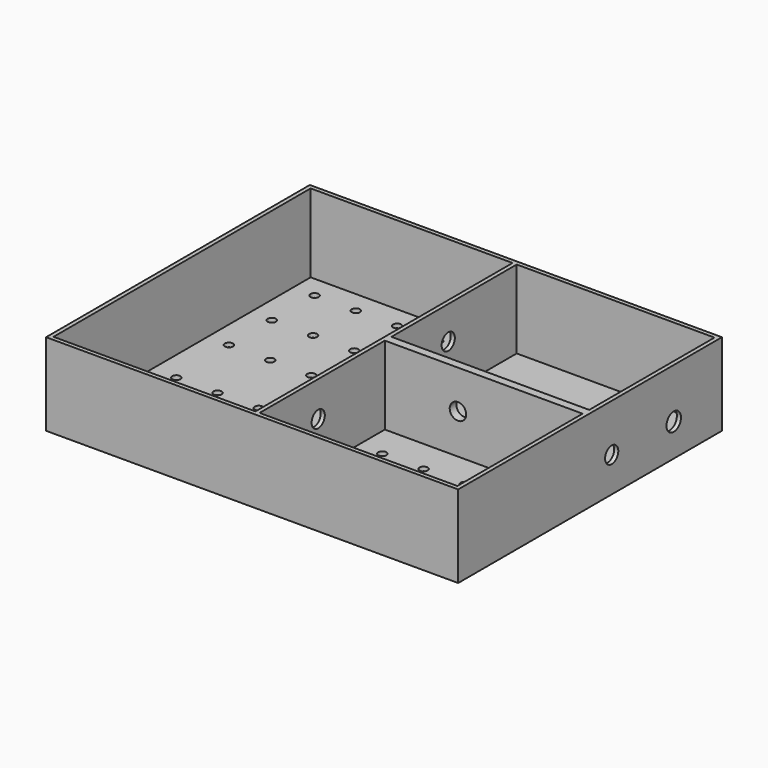
from build123d import *

# Parameters (mm, degrees)
F0_W      = 250
F0_H      = 200
F1_DEPTH  = 100
F2_T      = -5
F3_DEPTH  = 100
F4_T      = -5
F5_DEPTH  = 100
F6_T      = -5
F8_R      = 10
F9_DEPTH  = 25
F11_R     = 10
F12_DEPTH = 25
F14_R     = 5
F15_DEPTH = 25
F17_R     = 10
F18_DEPTH = 25
F19_R     = 11
F20_DEPTH = 25


# Not quite as in the source:
# - a shell that OpenCascade refuses in one call is made with other operations: the cavity is built on its own and cut out


with BuildPart() as f1:
    # F0 (on Top) → F1 (new body)
    with BuildSketch(Plane.XY):
        with Locations((375, -300)):
            Rectangle(F0_W, F0_H)
    extrude(amount=F1_DEPTH)

    # F2
    f2_openings = [f1.faces().sort_by_distance(p)[0] for p in [
        (375, -300, 100),
    ]]
    offset(amount=F2_T, openings=f2_openings)



with BuildPart() as f3:
    # F0 (on Top) → F3 (new body)
    with BuildSketch(Plane.XY):
        with Locations((375, -100)):
            Rectangle(F0_W, F0_H)
    extrude(amount=F3_DEPTH)

    # F4
    f4_openings = [f3.faces().sort_by_distance(p)[0] for p in [
        (375, -100, 100),
    ]]
    offset(amount=F4_T, openings=f4_openings)


with BuildPart() as f1_1:
    add(f1.part)

    add(f3.part)  # F5 merges F3
    # F0 (on Top) → F5 (join)
    with BuildSketch(Plane.XY):
        Polygon((250, 0), (0, 0), (0, -400), (250, -400), (250, -200), align=None)
    extrude(amount=F5_DEPTH)

    # F6: a shell. OpenCascade refuses it in one call, so the cavity is built on its own and cut out:
    # the body offset inwards by the wall thickness, plus a prism from it out through each open face.
    f6_core = offset(f1_1.part, amount=F6_T, kind=Kind.INTERSECTION, mode=Mode.PRIVATE)
    f6_exits = [f6_core.faces().sort_by_distance(p)[0] for p in [
        (127.5, -200, 95),
    ]]
    add(f6_core, mode=Mode.SUBTRACT)
    extrude(f6_exits, amount=-F6_T, mode=Mode.SUBTRACT)

    # F8 (on offset) → F9 (cut)
    with BuildSketch(Plane.YZ.offset(255)):
        with Locations((-108.8187620044, 59.8489716649)):
            Circle(F8_R)
        with Locations((-306.0356080532, 57.3764517903)):
            Circle(F8_R)
    extrude(amount=-F9_DEPTH, mode=Mode.SUBTRACT)

    # F11 (on offset) → F12 (cut)
    with BuildSketch(Plane.XZ.offset(205)):
        with Locations((343.7326848507, 53.2198026776)):
            Circle(F11_R)
    extrude(amount=-F12_DEPTH, mode=Mode.SUBTRACT)

    # F14 (on offset) → F15 (cut)
    with BuildSketch(Plane(origin=(0, 0, 0), x_dir=(1, 0, 0), z_dir=(0, 0, -1))):
        with Locations((31.2694571912, 31.7409522831)):
            Circle(F14_R)
        with Locations((484.199821949, 379.2208731174)):
            Circle(F14_R)
        with Locations((484.199821949, 312.2208731174)):
            Circle(F14_R)
        with Locations((484.199821949, 245.2208731174)):
            Circle(F14_R)
        with Locations((434.199821949, 379.2208731174)):
            Circle(F14_R)
        with Locations((434.199821949, 312.2208731174)):
            Circle(F14_R)
        with Locations((434.199821949, 245.2208731174)):
            Circle(F14_R)
        with Locations((384.199821949, 379.2208731174)):
            Circle(F14_R)
        with Locations((384.199821949, 312.2208731174)):
            Circle(F14_R)
        with Locations((384.199821949, 245.2208731174)):
            Circle(F14_R)
        with Locations((334.199821949, 379.2208731174)):
            Circle(F14_R)
        with Locations((334.199821949, 312.2208731174)):
            Circle(F14_R)
        with Locations((334.199821949, 245.2208731174)):
            Circle(F14_R)
        with Locations((284.199821949, 379.2208731174)):
            Circle(F14_R)
        with Locations((284.199821949, 312.2208731174)):
            Circle(F14_R)
        with Locations((284.199821949, 245.2208731174)):
            Circle(F14_R)
        with Locations((234.199821949, 379.2208731174)):
            Circle(F14_R)
        with Locations((234.199821949, 312.2208731174)):
            Circle(F14_R)
        with Locations((234.199821949, 245.2208731174)):
            Circle(F14_R)
        with Locations((184.199821949, 379.2208731174)):
            Circle(F14_R)
        with Locations((184.199821949, 312.2208731174)):
            Circle(F14_R)
        with Locations((184.199821949, 245.2208731174)):
            Circle(F14_R)
        with Locations((134.199821949, 379.2208731174)):
            Circle(F14_R)
        with Locations((134.199821949, 312.2208731174)):
            Circle(F14_R)
        with Locations((134.199821949, 245.2208731174)):
            Circle(F14_R)
        with Locations((84.199821949, 379.2208731174)):
            Circle(F14_R)
        with Locations((84.199821949, 312.2208731174)):
            Circle(F14_R)
        with Locations((84.199821949, 245.2208731174)):
            Circle(F14_R)
        with Locations((34.199821949, 379.2208731174)):
            Circle(F14_R)
        with Locations((34.199821949, 312.2208731174)):
            Circle(F14_R)
        with Locations((34.199821949, 245.2208731174)):
            Circle(F14_R)
        with Locations((31.2694571912, 96.7409522831)):
            Circle(F14_R)
        with Locations((31.2694571912, 161.7409522831)):
            Circle(F14_R)
        with Locations((81.2694571912, 31.7409522831)):
            Circle(F14_R)
        with Locations((81.2694571912, 96.7409522831)):
            Circle(F14_R)
        with Locations((81.2694571912, 161.7409522831)):
            Circle(F14_R)
        with Locations((131.2694571912, 31.7409522831)):
            Circle(F14_R)
        with Locations((131.2694571912, 96.7409522831)):
            Circle(F14_R)
        with Locations((131.2694571912, 161.7409522831)):
            Circle(F14_R)
        with Locations((181.2694571912, 31.7409522831)):
            Circle(F14_R)
        with Locations((181.2694571912, 96.7409522831)):
            Circle(F14_R)
        with Locations((181.2694571912, 161.7409522831)):
            Circle(F14_R)
        with Locations((231.2694571912, 31.7409522831)):
            Circle(F14_R)
        with Locations((231.2694571912, 96.7409522831)):
            Circle(F14_R)
        with Locations((231.2694571912, 161.7409522831)):
            Circle(F14_R)
    extrude(amount=-F15_DEPTH, mode=Mode.SUBTRACT)

    # F17 (on offset) → F18 (cut)
    with BuildSketch(Plane.YZ.offset(500)):
        with Locations((-167.1500247407, 42.3277354766)):
            Circle(F17_R)
    extrude(amount=-F18_DEPTH, mode=Mode.SUBTRACT)

    # F19 (on offset) → F20 (cut)
    with BuildSketch(Plane.YZ.offset(500)):
        with Locations((-73.0835795403, 39.550870657)):
            Circle(F19_R)
    extrude(amount=-F20_DEPTH, mode=Mode.SUBTRACT)


solid = f1_1.part
